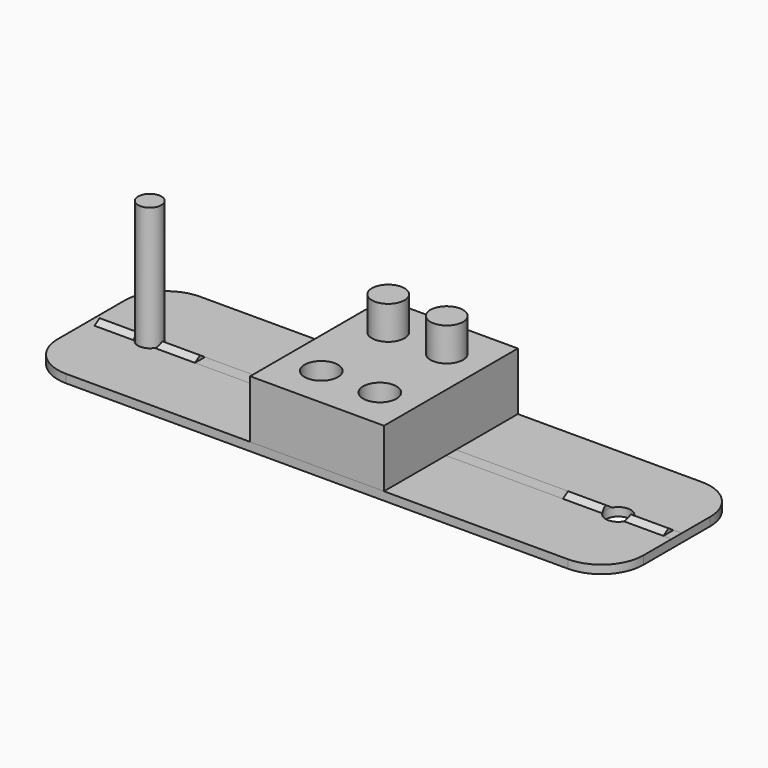
from build123d import *
from build123d import SkipClean  # not in build123d's __all__

# Parameters (mm, degrees)
F0_W      = 70
F0_H      = 20
F1_DEPTH  = 1
F3_D      = 3
F4_R      = 5
F7_DEPTH  = 0.5
F9_DEPTH  = 69.001
F10_W     = 16
F10_H     = 9.25
F10_H_2   = 1.5
F11_DEPTH = 6.9
F12_R     = 1.95
F13_DEPTH = 4
F14_R     = 2
F15_DEPTH = 4.2
F16_R     = 1.5
F17_DEPTH = 1
F18_R     = 1.4
F19_DEPTH = 14.8


with BuildPart() as f1:
    # F0 (on Top) → F1 (new body)
    with BuildSketch(Plane.XY):
        Rectangle(F0_W, F0_H)
    extrude(amount=F1_DEPTH)

    # F3 (through all)
    with Locations(Plane.XY.offset(1)):
        with Locations((-28, 0), (28, 0)):
            Hole(F3_D / 2)

    # F4
    f4_edges = [f1.edges().sort_by_distance(p)[0] for p in [
        (-35, 10, 0.5),
        (-35, -10, 0.5),
        (35, 10, 0.5),
        (35, -10, 0.5),
    ]]
    fillet(f4_edges, radius=F4_R)

    # F5 (on face) + F6 (on face) → F7 (join)
    with BuildSketch(Plane.XY.offset(1)):
        with BuildLine():
            Line((-29.2990381057, 0.75), (-34, 0.75))
            Line((-34, 0.75), (-34, -0.75))
            Line((-34, -0.75), (-29.2990381057, -0.75))
            ThreePointArc((-29.2990381057, -0.75), (-29.5, 0), (-29.2990381057, 0.75))
        make_face()
        with BuildLine():
            Line((-22, 0.75), (-26.7009618943, 0.75))
            ThreePointArc((-26.7009618943, 0.75), (-26.5511112606, 0.3882285677), (-26.5, 0))
            ThreePointArc((-26.5, 0), (-26.5511112606, -0.3882285677), (-26.7009618943, -0.75))
            Line((-26.7009618943, -0.75), (-22, -0.75))
            Line((-22, -0.75), (-22, 0.75))
        make_face()
    with BuildSketch(Plane.XY.offset(1)):
        with BuildLine():
            Line((26.7009618943, 0.75), (22, 0.75))
            Line((22, 0.75), (22, -0.75))
            Line((22, -0.75), (26.7009618943, -0.75))
            ThreePointArc((26.7009618943, -0.75), (26.5, 0), (26.7009618943, 0.75))
        make_face()
        with BuildLine():
            Line((34, 0.75), (29.2990381057, 0.75))
            ThreePointArc((29.2990381057, 0.75), (29.4488887394, 0.3882285677), (29.5, 0))
            ThreePointArc((29.5, 0), (29.4488887394, -0.3882285677), (29.2990381057, -0.75))
            Line((29.2990381057, -0.75), (34, -0.75))
            Line((34, -0.75), (34, 0.75))
        make_face()
    with SkipClean():  # cleaning this boolean's faces spoils the solid; the shape is the same uncleaned
        extrude(amount=F7_DEPTH)

    # F8 (on face) → F9 (cut, through all)
    with BuildSketch(Plane(origin=(-34, 0, 0), x_dir=(0, -1, 0), z_dir=(-1, 0, 0))):
        Polygon((-0.75, 1.5), (-0.75, 1), (0, 1.5), align=None)
        Polygon((0.75, 1.5), (0, 1.5), (0.75, 1), align=None)
    with SkipClean():  # cleaning this boolean's faces spoils the solid; the shape is the same uncleaned
        extrude(amount=-F9_DEPTH, mode=Mode.SUBTRACT)

    # F10 (on face) → F11 (join)
    with BuildSketch(Plane.XY.offset(1)):
        with Locations((0, -5.375)):
            Rectangle(F10_W, F10_H)
        Rectangle(F10_W, F10_H_2)
        with Locations((0, 5.375)):
            Rectangle(F10_W, F10_H)
    with SkipClean():  # cleaning this boolean's faces spoils the solid; the shape is the same uncleaned
        extrude(amount=F11_DEPTH)

    # F12 (on face) → F13 (join)
    with BuildSketch(Plane.XY.offset(7.9)):
        with Locations((-3.5, 5)):
            Circle(F12_R)
        with Locations((3.5, 5)):
            Circle(F12_R)
    with SkipClean():  # cleaning this boolean's faces spoils the solid; the shape is the same uncleaned
        extrude(amount=F13_DEPTH)

    # F14 (on face) → F15 (cut)
    with BuildSketch(Plane.XY.offset(7.9)):
        with Locations((-3.5, -5)):
            Circle(F14_R)
        with Locations((3.5, -5)):
            Circle(F14_R)
    with SkipClean():  # cleaning this boolean's faces spoils the solid; the shape is the same uncleaned
        extrude(amount=-F15_DEPTH, mode=Mode.SUBTRACT)

    # F16 (on face) → F17 (join)
    with BuildSketch(Plane.XY.offset(1)):
        with Locations((-28, 0)):
            Circle(F16_R)
    with SkipClean():  # cleaning this boolean's faces spoils the solid; the shape is the same uncleaned
        extrude(amount=-F17_DEPTH)

    # F18 (on face) → F19 (join)
    with BuildSketch(Plane.XY.offset(1)):
        with Locations((-28, 0)):
            Circle(F18_R)
    with SkipClean():  # cleaning this boolean's faces spoils the solid; the shape is the same uncleaned
        extrude(amount=F19_DEPTH)


solid = f1.part
